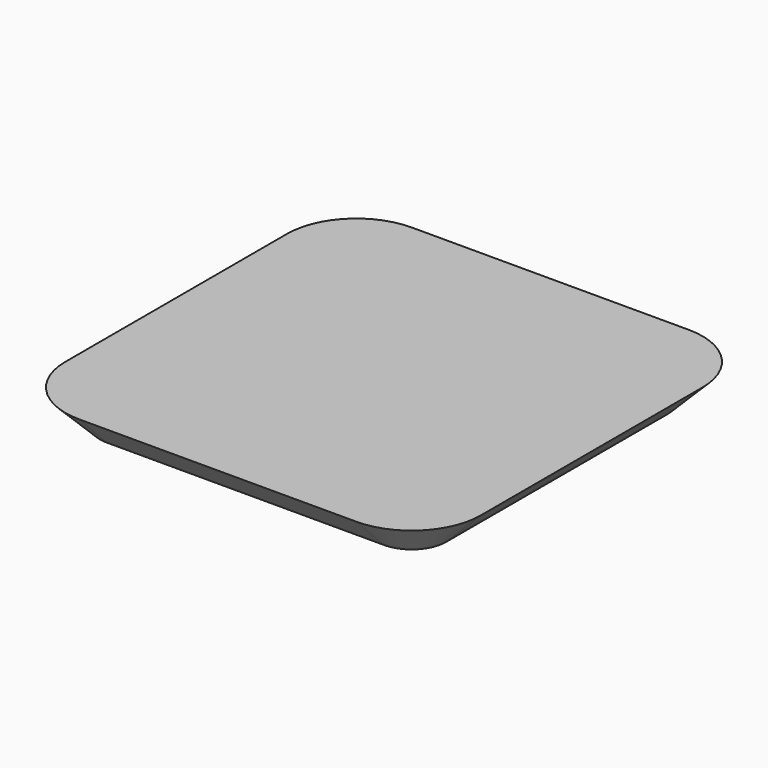
from build123d import *

# Parameters (mm, degrees)
F1_DEPTH = 10
F2_SIZE  = 9.99999


# Not quite as in the source:
# - a fillet or chamfer is up to 0.001 mm smaller than in the source, because OpenCascade refuses the exact size


with BuildPart() as f1:
    # F0 (on Top) → F1 (new body)
    with BuildSketch(Plane.XY):
        with BuildLine():
            Line((-40, -60), (40, -60))
            ThreePointArc((40, -60), (54.1421356237, -54.1421356237), (60, -40))
            Line((60, -40), (60, 40))
            ThreePointArc((60, 40), (54.1421356237, 54.1421356237), (40, 60))
            Line((40, 60), (-40, 60))
            ThreePointArc((-40, 60), (-54.1421356237, 54.1421356237), (-60, 40))
            Line((-60, 40), (-60, -40))
            ThreePointArc((-60, -40), (-54.1421356237, -54.1421356237), (-40, -60))
        make_face()
    extrude(amount=F1_DEPTH)

    # F2 (size 10 in the source; OpenCascade refuses exactly that, so slightly less here)
    f2_edges = [f1.edges().sort_by_distance(p)[0] for p in [
        (-60, 0, 0),
    ]]
    chamfer(f2_edges, length=F2_SIZE)


solid = f1.part
